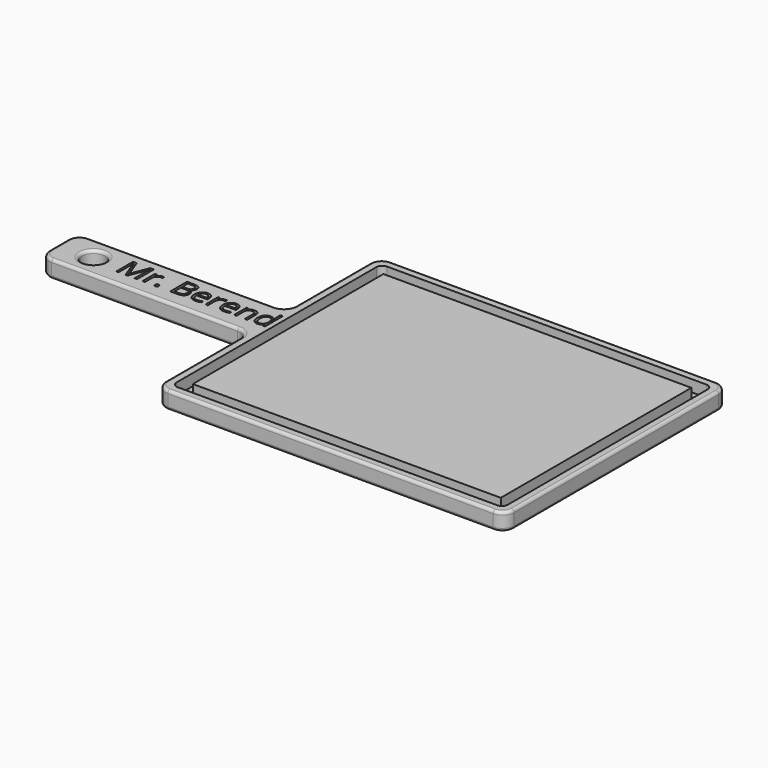
from build123d import *

# Parameters (mm, degrees)
F0_W         = 228.6
F0_H         = 50.8
F1_DEPTH     = 19.05
F2_R         = 12.7
F3_DEPTH     = 25.4
F5_R         = 12.7
F6_R         = 3.175
F7_W         = 336.55
F7_H         = 260.35
F8_DEPTH     = 12.7
F9_TEXT_SIZE = 32.1467733777
F10_DEPTH    = 3.175


# Not quite as in the source:
# - Text() gives the source's letters only with a copy of the font that has no kerning and outlines rounded to 1/6400 em; it was checked with that copy


with BuildPart() as f1:
    # F0 (on Top) → F1 (new body)
    with BuildSketch(Plane.XY):
        Polygon((0, 127), (0, 0), (381, 0), (381, 304.8), (0, 304.8), (0, 177.8), align=None)
        with Locations((-114.3, 152.4)):
            Rectangle(F0_W, F0_H)
    extrude(amount=F1_DEPTH)

    # F2 (on face) → F3 (cut)
    with BuildSketch(Plane.XY.offset(19.05)):
        with Locations((-190.5, 152.4)):
            Circle(F2_R)
    extrude(amount=-F3_DEPTH, mode=Mode.SUBTRACT)

    # F5
    f5_edges = [f1.edges().sort_by_distance(p)[0] for p in [
        (-228.6, 127, 9.525),
        (0, 127, 9.525),
        (0, 0, 9.525),
        (381, 0, 9.525),
        (381, 304.8, 9.525),
        (0, 304.8, 9.525),
        (0, 177.8, 9.525),
        (-228.6, 177.8, 9.525),
    ]]
    fillet(f5_edges, radius=F5_R)

    # F6
    f6_edges = [f1.edges().sort_by_distance(p)[0] for p in [
        (0, 63.5, 19.05),
        (-3.719744, 123.280256, 19.05),
        (3.719744, 3.719744, 19.05),
        (-114.3, 127, 19.05),
        (190.5, 0, 19.05),
        (-224.880256, 130.719744, 19.05),
        (377.280256, 3.719744, 19.05),
        (-228.6, 152.4, 19.05),
        (381, 152.4, 19.05),
        (-224.880256, 174.080256, 19.05),
        (377.280256, 301.080256, 19.05),
        (-114.3, 177.8, 19.05),
        (190.5, 304.8, 19.05),
        (-3.719744, 181.519744, 19.05),
        (3.719744, 301.080256, 19.05),
        (0, 241.3, 19.05),
        (-203.2, 152.4, 19.05),
        (0, 63.5, 0),
        (-3.719744, 123.280256, 0),
        (3.719744, 3.719744, 0),
        (-114.3, 127, 0),
        (190.5, 0, 0),
        (-224.880256, 130.719744, 0),
        (377.280256, 3.719744, 0),
        (-228.6, 152.4, 0),
        (381, 152.4, 0),
        (-224.880256, 174.080256, 0),
        (377.280256, 301.080256, 0),
        (-114.3, 177.8, 0),
        (190.5, 304.8, 0),
        (-3.719744, 181.519744, 0),
        (3.719744, 301.080256, 0),
        (0, 241.3, 0),
        (-203.2, 152.4, 0),
    ]]
    fillet(f6_edges, radius=F6_R)

    # F7 (on face) → F8 (cut)
    with BuildSketch(Plane.XY.offset(19.05)):
        with BuildLine():
            Line((365.125, 295.275), (15.875, 295.275))
            ThreePointArc((15.875, 295.275), (11.3848719395, 293.4151280605), (9.525, 288.925))
            Line((9.525, 288.925), (9.525, 15.875))
            ThreePointArc((9.525, 15.875), (11.3848719395, 11.3848719395), (15.875, 9.525))
            Line((15.875, 9.525), (365.125, 9.525))
            ThreePointArc((365.125, 9.525), (369.6151280605, 11.3848719395), (371.475, 15.875))
            Line((371.475, 15.875), (371.475, 288.925))
            ThreePointArc((371.475, 288.925), (369.6151280605, 293.4151280605), (365.125, 295.275))
        make_face()
        with Locations((190.5, 152.4)):
            Rectangle(F7_W, F7_H, mode=Mode.SUBTRACT)
    extrude(amount=-F8_DEPTH, mode=Mode.SUBTRACT)

    # F9 (on face) → F10 (cut)
    with BuildSketch(Plane.XY.offset(19.05)):
        with Locations((-161.925, 143.8593231681)):
            Text('Mr. Berend', F9_TEXT_SIZE, font='Open Sans', text_align=(TextAlign.LEFT, TextAlign.BOTTOM))
    extrude(amount=-F10_DEPTH, mode=Mode.SUBTRACT)


solid = f1.part
